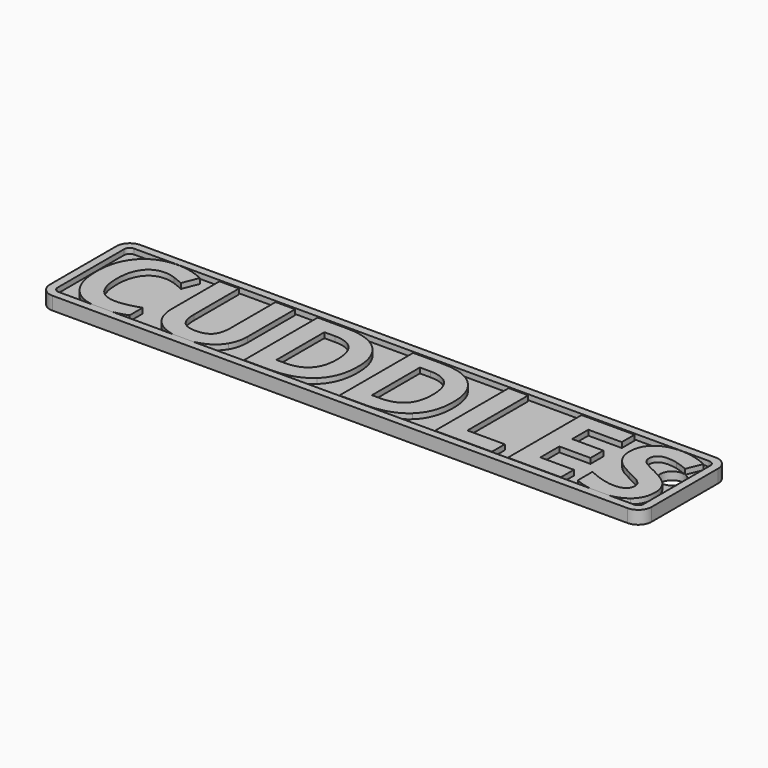
from build123d import *

# Parameters (mm, degrees)
F1_DEPTH      = 3
F2_W          = 229.4094786048
F2_H          = 41.8851505965
F3_DEPTH      = 2
F3_DEPTH_BACK = 3
F4_R          = 5.08
F5_T          = -3
F6_R          = 4.561092178
F7_DEPTH      = 2.0010001
F7_DEPTH_BACK = 3.001


with BuildPart() as f1:
    # F0 (on Top) → F1 (new body)
    with BuildSketch(Plane.XY):
        with BuildLine():
            add(Edge.make_bspline(
                [(-93.9181388467, -17.3174301162), (-96.4073282749, -17.8015217971), (-99.1684330301, -17.8015217971)],
                knots=[0.4822306436, 0.4822306436, 0.4822306436, 1, 1, 1], degree=2))
            Line((-93.9181388467, -17.3174301162), (-103.7374619259, -17.3174301162))
            add(Edge.make_bspline(
                [(-99.1684330301, -17.8015217971), (-101.6405830138, -17.8015217971), (-103.7374619259, -17.3174301162)],
                knots=[0, 0, 0, 0.3226952609, 0.3226952609, 0.3226952609], degree=2))
        make_face()
        with BuildLine():
            add(Edge.make_bspline(
                [(-101.3807325462, 18.0904185399), (-99.9833916771, 18.2902024082), (-98.4691894911, 18.2902024082)],
                knots=[0.6982247505, 0.6982247505, 0.6982247505, 1, 1, 1], degree=2))
            Line((-101.3807325462, 18.0904185399), (-95.5563073813, 18.0904185399))
            add(Edge.make_bspline(
                [(-98.4691894911, 18.2902024082), (-97.014926765, 18.2902024082), (-95.5563073813, 18.0904185399)],
                knots=[0, 0, 0, 0.2845995164, 0.2845995164, 0.2845995164], degree=2))
        make_face()
        with BuildLine():
            add(Edge.make_bspline(
                [(-63.4014608269, -17.3174301162), (-65.5283772477, -17.8015217971), (-68.0252015623, -17.8015217971)],
                knots=[0.4435987872, 0.4435987872, 0.4435987872, 1, 1, 1], degree=2))
            Line((-63.4014608269, -17.3174301162), (-72.6584475841, -17.3174301162))
            add(Edge.make_bspline(
                [(-68.0252015623, -17.8015217971), (-70.5525436843, -17.8015217971), (-72.6584475841, -17.3174301162)],
                knots=[0, 0, 0, 0.3733370206, 0.3733370206, 0.3733370206], degree=2))
        make_face()
        Polygon((27.9402111693, 17.7907427375), (27.9402111693, -17.3174301162), (49.6244448732, -17.3174301162), (49.6244448732, -11.170234169), (35.3860022604, -11.170234169), (35.3860022604, 17.7907427375), align=None)
        Polygon((55.7255368508, 17.7907427375), (55.7255368508, -17.3174301162), (75.9421275224, -17.3174301162), (75.9421275224, -11.170234169), (63.1713279419, -11.170234169), (63.1713279419, -2.1184881367), (75.0584681049, -2.1184881367), (75.0584681049, 3.982603841), (63.1713279419, 3.982603841), (63.1713279419, 11.6896507599), (75.9421275224, 11.6896507599), (75.9421275224, 17.7907427375), align=None)
        with BuildLine():
            Line((95.7000665404, -17.3174301162), (85.9724620363, -17.3174301162))
            add(Edge.make_bspline(
                [(91.0488615627, -17.8015217971), (88.3615755935, -17.8015217971), (85.9724620363, -17.3174301162)],
                knots=[0, 0, 0, 0.477766543, 0.477766543, 0.477766543], degree=2))
            add(Edge.make_bspline(
                [(95.7000665404, -17.3174301162), (93.6103993378, -17.8015217971), (91.0488615627, -17.8015217971)],
                knots=[0.5796214889, 0.5796214889, 0.5796214889, 1, 1, 1], degree=2))
        make_face()
        with BuildLine():
            add(Edge.make_bspline(
                [(90.5291697988, 18.0904185399), (91.8741443448, 18.2902024082), (93.4001640126, 18.2902024082)],
                knots=[0.7260728655, 0.7260728655, 0.7260728655, 1, 1, 1], degree=2))
            Line((90.5291697988, 18.0904185399), (96.3666525375, 18.0904185399))
            add(Edge.make_bspline(
                [(93.4001640126, 18.2902024082), (94.92205694, 18.2902024082), (96.3666525375, 18.0904185399)],
                knots=[0, 0, 0, 0.5563486403, 0.5563486403, 0.5563486403], degree=2))
        make_face()
        with BuildLine():
            Line((-72.6584475841, -17.3174301162), (-63.4014608269, -17.3174301162))
            add(Edge.make_bspline(
                [(-60.2451566916, -16.237828828), (-61.7057464338, -16.9314811327), (-63.4014608269, -17.3174301162)],
                knots=[0, 0, 0, 0.4435987872, 0.4435987872, 0.4435987872], degree=2))
            add(Edge.make_bspline(
                [(-55.2121400097, -11.746533789), (-56.9525648623, -14.6741358589), (-60.2451566916, -16.237828828)],
                knots=[0, 0, 0, 1, 1, 1], degree=2))
            add(Edge.make_bspline(
                [(-53.4717151572, -4.9231462876), (-53.4717151572, -8.8189317192), (-55.2121400097, -11.746533789)],
                knots=[0, 0, 0, 1, 1, 1], degree=2))
            Line((-53.4717151572, -4.9231462876), (-53.4717151572, 17.7907427375))
            Line((-53.4717151572, 17.7907427375), (-60.8944542635, 17.7907427375))
            Line((-60.8944542635, 17.7907427375), (-60.8944542635, -3.6552871235))
            add(Edge.make_bspline(
                [(-62.5388291794, -9.6449611746), (-60.8944542635, -7.7354884335), (-60.8944542635, -3.6552871235)],
                knots=[0, 0, 0, 1, 1, 1], degree=2))
            add(Edge.make_bspline(
                [(-67.8331016889, -11.5544339157), (-64.1832040953, -11.5544339157), (-62.5388291794, -9.6449611746)],
                knots=[0, 0, 0, 1, 1, 1], degree=2))
            add(Edge.make_bspline(
                [(-73.2387921251, -9.656487167), (-71.6059432016, -11.5544339157), (-67.8331016889, -11.5544339157)],
                knots=[0, 0, 0, 1, 1, 1], degree=2))
            add(Edge.make_bspline(
                [(-74.8716410486, -3.7013910931), (-74.8716410486, -7.7585404183), (-73.2387921251, -9.656487167)],
                knots=[0, 0, 0, 1, 1, 1], degree=2))
            Line((-74.8716410486, -3.7013910931), (-74.8716410486, 17.7907427375))
            Line((-74.8716410486, 17.7907427375), (-82.2866961599, 17.7907427375))
            Line((-82.2866961599, 17.7907427375), (-82.2866961599, -4.8309383484))
            add(Edge.make_bspline(
                [(-78.5407486296, -14.3283560869), (-82.2866961599, -10.8551903767), (-82.2866961599, -4.8309383484)],
                knots=[0, 0, 0, 1, 1, 1], degree=2))
            add(Edge.make_bspline(
                [(-72.6584475841, -17.3174301162), (-76.1933019896, -16.5048604587), (-78.5407486296, -14.3283560869)],
                knots=[0.3733370206, 0.3733370206, 0.3733370206, 1, 1, 1], degree=2))
        make_face()
        with BuildLine():
            Line((-44.873324826, 17.7907427375), (-44.873324826, -17.3174301162))
            Line((-44.873324826, -17.3174301162), (-34.9302353813, -17.3174301162))
            add(Edge.make_bspline(
                [(-20.6802667761, -12.7070331558), (-25.6172335212, -17.3174301162), (-34.9302353813, -17.3174301162)],
                knots=[0, 0, 0, 1, 1, 1], degree=2))
            add(Edge.make_bspline(
                [(-15.7433000309, 0.5709100903), (-15.7433000309, -8.0966361954), (-20.6802667761, -12.7070331558)],
                knots=[0, 0, 0, 1, 1, 1], degree=2))
            add(Edge.make_bspline(
                [(-20.4996928951, 13.2533437289), (-15.7433000309, 8.7159447204), (-15.7433000309, 0.5709100903)],
                knots=[0, 0, 0, 1, 1, 1], degree=2))
            add(Edge.make_bspline(
                [(-33.8544760905, 17.7907427375), (-25.2560857593, 17.7907427375), (-20.4996928951, 13.2533437289)],
                knots=[0, 0, 0, 1, 1, 1], degree=2))
            Line((-33.8544760905, 17.7907427375), (-44.873324826, 17.7907427375))
        make_face()
        with BuildLine():
            add(Edge.make_bspline(
                [(-23.4810829295, 0.3788102169), (-23.4810829295, 11.6896507599), (-33.4702763438, 11.6896507599)],
                knots=[0, 0, 0, 1, 1, 1], degree=2))
            add(Edge.make_bspline(
                [(-34.2386758372, -11.170234169), (-23.4810829295, -11.170234169), (-23.4810829295, 0.3788102169)],
                knots=[0, 0, 0, 1, 1, 1], degree=2))
            Line((-34.2386758372, -11.170234169), (-37.4275337348, -11.170234169))
            Line((-37.4275337348, -11.170234169), (-37.4275337348, 11.6896507599))
            Line((-37.4275337348, 11.6896507599), (-33.4702763438, 11.6896507599))
        make_face(mode=Mode.SUBTRACT)
        with BuildLine():
            Line((-8.4665568284, 17.7907427375), (-8.4665568284, -17.3174301162))
            Line((-8.4665568284, -17.3174301162), (1.4765326163, -17.3174301162))
            add(Edge.make_bspline(
                [(15.7265012216, -12.7070331558), (10.7895344764, -17.3174301162), (1.4765326163, -17.3174301162)],
                knots=[0, 0, 0, 1, 1, 1], degree=2))
            add(Edge.make_bspline(
                [(20.6634679667, 0.5709100903), (20.6634679667, -8.0966361954), (15.7265012216, -12.7070331558)],
                knots=[0, 0, 0, 1, 1, 1], degree=2))
            add(Edge.make_bspline(
                [(15.9070751025, 13.2533437289), (20.6634679667, 8.7159447204), (20.6634679667, 0.5709100903)],
                knots=[0, 0, 0, 1, 1, 1], degree=2))
            add(Edge.make_bspline(
                [(2.5522919071, 17.7907427375), (11.1506822383, 17.7907427375), (15.9070751025, 13.2533437289)],
                knots=[0, 0, 0, 1, 1, 1], degree=2))
            Line((2.5522919071, 17.7907427375), (-8.4665568284, 17.7907427375))
        make_face()
        with BuildLine():
            add(Edge.make_bspline(
                [(12.9256850681, 0.3788102169), (12.9256850681, 11.6896507599), (2.9364916538, 11.6896507599)],
                knots=[0, 0, 0, 1, 1, 1], degree=2))
            add(Edge.make_bspline(
                [(2.1680921604, -11.170234169), (12.9256850681, -11.170234169), (12.9256850681, 0.3788102169)],
                knots=[0, 0, 0, 1, 1, 1], degree=2))
            Line((2.1680921604, -11.170234169), (-1.0207657372, -11.170234169))
            Line((-1.0207657372, -11.170234169), (-1.0207657372, 11.6896507599))
            Line((-1.0207657372, 11.6896507599), (2.9364916538, 11.6896507599))
        make_face(mode=Mode.SUBTRACT)
        with BuildLine():
            add(Edge.make_bspline(
                [(85.9724620363, -17.3174301162), (83.36098777, -16.7882828251), (81.1057721181, -15.6807391953)],
                knots=[0.477766543, 0.477766543, 0.477766543, 1, 1, 1], degree=2))
            Line((85.9724620363, -17.3174301162), (95.7000665404, -17.3174301162))
            add(Edge.make_bspline(
                [(100.5654892886, -15.0621776031), (98.5813175641, -16.6499603635), (95.7000665404, -17.3174301162)],
                knots=[0, 0, 0, 0.5796214889, 0.5796214889, 0.5796214889], degree=2))
            add(Edge.make_bspline(
                [(103.9887090317, -7.5664405449), (103.9887090317, -12.3228334091), (100.5654892886, -15.0621776031)],
                knots=[0, 0, 0, 1, 1, 1], degree=2))
            add(Edge.make_bspline(
                [(102.1637602349, -1.7688663672), (103.9887090317, -4.1316948094), (103.9887090317, -7.5664405449)],
                knots=[0, 0, 0, 1, 1, 1], degree=2))
            add(Edge.make_bspline(
                [(95.4133706853, 2.9529485198), (100.338811438, 0.5939620751), (102.1637602349, -1.7688663672)],
                knots=[0, 0, 0, 1, 1, 1], degree=2))
            add(Edge.make_bspline(
                [(90.6992397932, 5.4118268987), (91.6943171372, 4.7279513496), (95.4133706853, 2.9529485198)],
                knots=[0, 0, 0, 1, 1, 1], degree=2))
            add(Edge.make_bspline(
                [(89.2469647507, 6.8295239641), (89.7041624493, 6.0957024479), (90.6992397932, 5.4118268987)],
                knots=[0, 0, 0, 1, 1, 1], degree=2))
            add(Edge.make_bspline(
                [(88.7897670521, 8.5468968318), (88.7897670521, 7.5633454803), (89.2469647507, 6.8295239641)],
                knots=[0, 0, 0, 1, 1, 1], degree=2))
            add(Edge.make_bspline(
                [(89.9193143074, 11.1133511398), (88.7897670521, 10.1297997882), (88.7897670521, 8.5468968318)],
                knots=[0, 0, 0, 1, 1, 1], degree=2))
            add(Edge.make_bspline(
                [(93.1619601696, 12.0969024914), (91.0488615627, 12.0969024914), (89.9193143074, 11.1133511398)],
                knots=[0, 0, 0, 1, 1, 1], degree=2))
            add(Edge.make_bspline(
                [(96.7734377886, 11.6397047928), (94.9369629994, 12.0969024914), (93.1619601696, 12.0969024914)],
                knots=[0, 0, 0, 1, 1, 1], degree=2))
            add(Edge.make_bspline(
                [(101.4222547237, 10.0299078541), (98.6099125779, 11.1825070942), (96.7734377886, 11.6397047928)],
                knots=[0, 0, 0, 1, 1, 1], degree=2))
            Line((101.4222547237, 10.0299078541), (103.8196611432, 15.8236400344))
            add(Edge.make_bspline(
                [(98.6214385703, 17.6447468338), (101.1072109314, 16.9992912593), (103.8196611432, 15.8236400344)],
                knots=[0, 0, 0, 1, 1, 1], degree=2))
            add(Edge.make_bspline(
                [(96.3666525375, 18.0904185399), (97.5186222822, 17.931104077), (98.6214385703, 17.6447468338)],
                knots=[0.5563486403, 0.5563486403, 0.5563486403, 1, 1, 1], degree=2))
            Line((96.3666525375, 18.0904185399), (90.5291697988, 18.0904185399))
            add(Edge.make_bspline(
                [(84.6711457675, 15.6276981636), (86.9641723979, 17.5608702498), (90.5291697988, 18.0904185399)],
                knots=[0, 0, 0, 0.7260728655, 0.7260728655, 0.7260728655], degree=2))
            add(Edge.make_bspline(
                [(81.5130238496, 8.3010089939), (81.5130238496, 12.9651939189), (84.6711457675, 15.6276981636)],
                knots=[0, 0, 0, 1, 1, 1], degree=2))
            add(Edge.make_bspline(
                [(82.4735232163, 3.982603841), (81.5130238496, 5.8344466201), (81.5130238496, 8.3010089939)],
                knots=[0, 0, 0, 1, 1, 1], degree=2))
            add(Edge.make_bspline(
                [(85.0438195218, 0.7399579788), (83.4340225831, 2.1307610619), (82.4735232163, 3.982603841)],
                knots=[0, 0, 0, 1, 1, 1], degree=2))
            add(Edge.make_bspline(
                [(89.8655263429, -2.1645921063), (86.6536164605, -0.6508451042), (85.0438195218, 0.7399579788)],
                knots=[0, 0, 0, 1, 1, 1], degree=2))
            add(Edge.make_bspline(
                [(94.4182933413, -4.5427885384), (93.3002720784, -3.8012830272), (89.8655263429, -2.1645921063)],
                knots=[0, 0, 0, 1, 1, 1], degree=2))
            add(Edge.make_bspline(
                [(96.1126142243, -6.0911135176), (95.5363146042, -5.2842940495), (94.4182933413, -4.5427885384)],
                knots=[0, 0, 0, 1, 1, 1], degree=2))
            add(Edge.make_bspline(
                [(96.6889138443, -7.9275883068), (96.6889138443, -6.8979329856), (96.1126142243, -6.0911135176)],
                knots=[0, 0, 0, 1, 1, 1], degree=2))
            add(Edge.make_bspline(
                [(95.3787927081, -10.7130364704), (96.6889138443, -9.7794310859), (96.6889138443, -7.9275883068)],
                knots=[0, 0, 0, 1, 1, 1], degree=2))
            add(Edge.make_bspline(
                [(91.6251611828, -11.6466418549), (94.0686715718, -11.6466418549), (95.3787927081, -10.7130364704)],
                knots=[0, 0, 0, 1, 1, 1], degree=2))
            add(Edge.make_bspline(
                [(87.118498154, -11.0011862804), (89.5812185303, -11.6466418549), (91.6251611828, -11.6466418549)],
                knots=[0, 0, 0, 1, 1, 1], degree=2))
            add(Edge.make_bspline(
                [(81.1057721181, -8.7651437546), (84.6557777776, -10.355730706), (87.118498154, -11.0011862804)],
                knots=[0, 0, 0, 1, 1, 1], degree=2))
            Line((81.1057721181, -8.7651437546), (81.1057721181, -15.6807391953))
        make_face()
        with BuildLine():
            Line((-103.7374619259, -17.3174301162), (-93.9181388467, -17.3174301162))
            add(Edge.make_bspline(
                [(-89.5173353929, -15.9957829876), (-91.5998026893, -16.8665655759), (-93.9181388467, -17.3174301162)],
                knots=[0, 0, 0, 0.4822306436, 0.4822306436, 0.4822306436], degree=2))
            Line((-89.5173353929, -15.9957829876), (-89.5173353929, -9.7563791011))
            add(Edge.make_bspline(
                [(-98.4691894911, -11.6005378853), (-94.7731879278, -11.6005378853), (-89.5173353929, -9.7563791011)],
                knots=[0, 0, 0, 1, 1, 1], degree=2))
            add(Edge.make_bspline(
                [(-107.2827316804, 0.140606374), (-107.2827316804, -11.6005378853), (-98.4691894911, -11.6005378853)],
                knots=[0, 0, 0, 1, 1, 1], degree=2))
            add(Edge.make_bspline(
                [(-104.9775332002, 8.9387805735), (-107.2827316804, 5.7806586556), (-107.2827316804, 0.140606374)],
                knots=[0, 0, 0, 1, 1, 1], degree=2))
            add(Edge.make_bspline(
                [(-98.4691894911, 12.0969024914), (-102.67233472, 12.0969024914), (-104.9775332002, 8.9387805735)],
                knots=[0, 0, 0, 1, 1, 1], degree=2))
            add(Edge.make_bspline(
                [(-94.5580360696, 11.4015009498), (-96.5481907576, 12.0969024914), (-98.4691894911, 12.0969024914)],
                knots=[0, 0, 0, 1, 1, 1], degree=2))
            add(Edge.make_bspline(
                [(-90.5930946837, 9.7686520263), (-92.5678813817, 10.7060994083), (-94.5580360696, 11.4015009498)],
                knots=[0, 0, 0, 1, 1, 1], degree=2))
            Line((-90.5930946837, 9.7686520263), (-88.1956882642, 15.8236400344))
            add(Edge.make_bspline(
                [(-95.5563073813, 18.0904185399), (-91.8897621051, 17.5882199495), (-88.1956882642, 15.8236400344)],
                knots=[0.2845995164, 0.2845995164, 0.2845995164, 1, 1, 1], degree=2))
            Line((-95.5563073813, 18.0904185399), (-101.3807325462, 18.0904185399))
            add(Edge.make_bspline(
                [(-107.221259721, 16.0964218546), (-104.6137941745, 17.6281737342), (-101.3807325462, 18.0904185399)],
                knots=[0, 0, 0, 0.6982247505, 0.6982247505, 0.6982247505], degree=2))
            add(Edge.make_bspline(
                [(-112.9496779443, 9.7840200162), (-110.9556812589, 13.9026413009), (-107.221259721, 16.0964218546)],
                knots=[0, 0, 0, 1, 1, 1], degree=2))
            add(Edge.make_bspline(
                [(-114.9436746297, 0.1867103436), (-114.9436746297, 5.6653987316), (-112.9496779443, 9.7840200162)],
                knots=[0, 0, 0, 1, 1, 1], degree=2))
            add(Edge.make_bspline(
                [(-110.8865253045, -13.152704862), (-114.9436746297, -8.5038879269), (-114.9436746297, 0.1867103436)],
                knots=[0, 0, 0, 1, 1, 1], degree=2))
            add(Edge.make_bspline(
                [(-103.7374619259, -17.3174301162), (-108.1385988393, -16.3013706033), (-110.8865253045, -13.152704862)],
                knots=[0.3226952609, 0.3226952609, 0.3226952609, 1, 1, 1], degree=2))
        make_face()
    extrude(amount=F1_DEPTH)


with BuildPart() as f3:
    # F2 (on face) → F3 (new body, two sides)
    with BuildSketch(Plane(origin=(0, 0, 0), x_dir=(1, 0, 0), z_dir=(0, 0, -1))) as f3_sk:
        with Locations((-5.7197250426, -0.4553580657)):
            Rectangle(F2_W, F2_H)
        with BuildLine():
            Line((-8.4665568284, -17.7907427375), (-8.4665568284, 17.3174301162))
            Line((-8.4665568284, 17.3174301162), (1.4765326163, 17.3174301162))
            add(Edge.make_bspline(
                [(1.4765326163, 17.3174301162), (10.7895344764, 17.3174301162), (20.6634679667, 8.0966361954), (20.6634679667, -8.7159447204), (11.1506822383, -17.7907427375), (2.5522919071, -17.7907427375)],
                knots=[0, 0, 0, 1, 2, 2.9397163121, 3.8794326241, 3.8794326241, 3.8794326241], degree=2))
            Line((2.5522919071, -17.7907427375), (-8.4665568284, -17.7907427375))
        make_face(mode=Mode.SUBTRACT)
        with BuildLine():
            Line((1.4765326163, 17.3174301162), (-8.4665568284, 17.3174301162))
            Line((-8.4665568284, 17.3174301162), (-8.4665568284, -17.7907427375))
            Line((-8.4665568284, -17.7907427375), (2.5522919071, -17.7907427375))
            add(Edge.make_bspline(
                [(1.4765326163, 17.3174301162), (10.7895344764, 17.3174301162), (20.6634679667, 8.0966361954), (20.6634679667, -8.7159447204), (11.1506822383, -17.7907427375), (2.5522919071, -17.7907427375)],
                knots=[0, 0, 0, 1, 2, 2.9397163121, 3.8794326241, 3.8794326241, 3.8794326241], degree=2))
        make_face()
        with BuildLine():
            Line((2.9364916538, -11.6896507599), (-1.0207657372, -11.6896507599))
            Line((-1.0207657372, -11.6896507599), (-1.0207657372, 11.170234169))
            Line((-1.0207657372, 11.170234169), (2.1680921604, 11.170234169))
            add(Edge.make_bspline(
                [(2.9364916538, -11.6896507599), (12.9256850681, -11.6896507599), (12.9256850681, 11.170234169), (2.1680921604, 11.170234169)],
                knots=[0, 0, 0, 1, 2.0210597826, 2.0210597826, 2.0210597826], degree=2))
        make_face(mode=Mode.SUBTRACT)
        with BuildLine():
            Line((-1.0207657372, 11.170234169), (-1.0207657372, -11.6896507599))
            Line((-1.0207657372, -11.6896507599), (2.9364916538, -11.6896507599))
            add(Edge.make_bspline(
                [(2.9364916538, -11.6896507599), (12.9256850681, -11.6896507599), (12.9256850681, 11.170234169), (2.1680921604, 11.170234169)],
                knots=[0, 0, 0, 1, 2.0210597826, 2.0210597826, 2.0210597826], degree=2))
            Line((2.1680921604, 11.170234169), (-1.0207657372, 11.170234169))
        make_face()
    extrude(amount=F3_DEPTH)
    extrude(f3_sk.sketch, amount=-F3_DEPTH_BACK)

    # F4
    f4_edges = [f3.edges().sort_by_distance(p)[0] for p in [
        (-120.424464, 21.397933, 0.5),
        (-120.424464, -20.487217, 0.5),
        (108.985014, -20.487217, 0.5),
        (108.985014, 21.397933, 0.5),
    ]]
    fillet(f4_edges, radius=F4_R)

    # F5
    f5_openings = [f3.faces().sort_by_distance(p)[0] for p in [
        (-5.719725, 0.455358, 3),
    ]]
    offset(amount=F5_T, openings=f5_openings)


with BuildPart() as f7_tool:
    # F6 (on face) → F7 (new body, two sides)
    with BuildSketch(Plane.XY.offset(1)) as f7_sk:
        with Locations((99.8875945807, 5.7600070722)):
            Circle(F6_R)
    extrude(amount=F7_DEPTH)
    extrude(f7_sk.sketch, amount=-F7_DEPTH_BACK)


with BuildPart() as f1_1:
    add(f1.part)

    # F7: cut by f7_tool
    add(f7_tool.part, mode=Mode.SUBTRACT)


with BuildPart() as f3_1:
    add(f3.part)

    # F7: cut by f7_tool
    add(f7_tool.part, mode=Mode.SUBTRACT)


solid = Compound([f1_1.part, f3_1.part])
